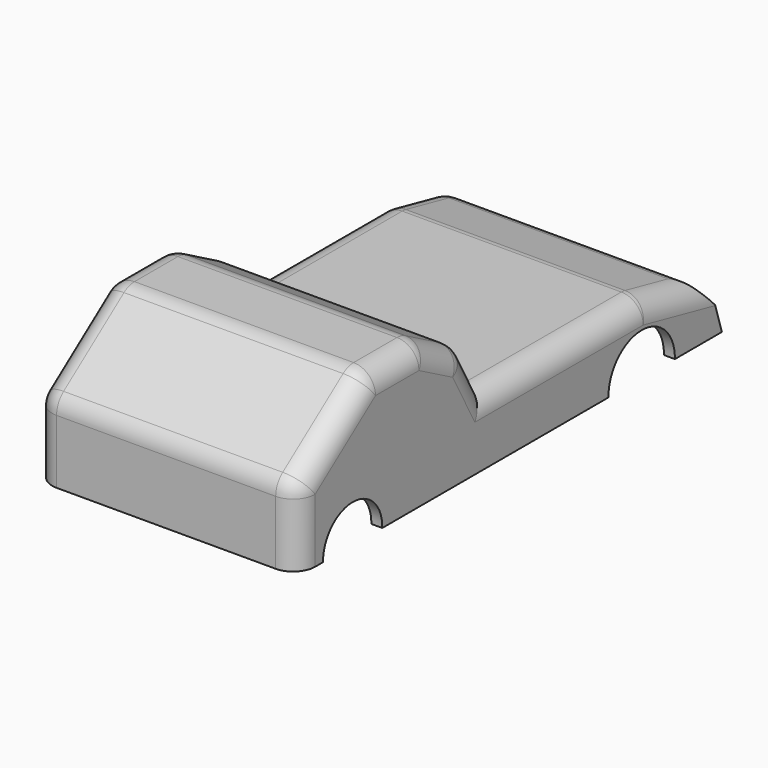
from build123d import *

# Parameters (mm, degrees)
F1_DEPTH      = 60
F2_T          = -2.5
F3_T1_DEPTH   = 31.5029107171
F3_T3_DEPTH   = 19.2704775269
F3_T5_DEPTH   = 59.0151251094
F3_T7_DEPTH   = 50
F3_T9_DEPTH   = 12.544705842
F3_T11_DEPTH  = 26.6507558857
F3_T13_DEPTH  = 10.9735782615
F3_T15_DEPTH  = 12.384029335
F3_T17_DEPTH  = 21.4746284083
F3_T19_DEPTH  = 27.0595039158
F3_T24_DEPTH  = 5
F3_T30_DEPTH  = 5
F3_T36_DEPTH  = 5
F3_T42_DEPTH  = 5
F3_T48_DEPTH  = 5
F3_T54_DEPTH  = 5
F3_T60_DEPTH  = 5
F3_T66_DEPTH  = 5
F3_T72_DEPTH  = 5
F3_T78_DEPTH  = 5
F3_T84_DEPTH  = 5
F3_T90_DEPTH  = 57.5475311177
F3_T95_DEPTH  = 22.7575976563
F3_T100_DEPTH = 57.5475311177
F3_T105_DEPTH = 22.7575976563
F3_T111_DEPTH = 22.7575976563
F3_T115_DEPTH = 57.5475311177
F3_T122_DEPTH = 57.5475311177
F3_T126_DEPTH = 22.7575976563
F4_R          = 8.968677233
F4_R_2        = 8.5168287605
F5_DEPTH      = 60
F6_R          = 9.472590991
F6_R_2        = 8.4503132789
F7_DEPTH      = 65.4


# Not quite as in the source:
# - a fillet or chamfer that OpenCascade refuses, or shapes differently, is made with other operations: its cross-section is extruded or revolved along the edge and cut away or added


with BuildPart() as f1:
    # F0 (on Right) → F1 (new body)
    with BuildSketch(Plane.YZ):
        Polygon((-44.8060370982, 22.3060343415), (-65.3663799167, 6.9827586412), (-65.3663799167, -10.0862076506), (55.6681081653, -10.0862076506), (53.7284500897, -3.8793103304), (48.1034480035, 2.3275862914), (33.7500013411, 5.4310346022), (20.5603465438, 5.4310346022), (4.4612074271, 5.4310346022), (-11.8318963796, 5.4310346022), (-17.4568966031, 15.7112069428), (-29.4827595353, 22.3060343415), align=None)
    extrude(amount=F1_DEPTH)

    # F2
    f2_openings = [f1.faces().sort_by_distance(p)[0] for p in [
        (30, -4.849136, -10.086208),
    ]]
    offset(amount=F2_T, openings=f2_openings, kind=Kind.INTERSECTION)

    # F3: fillet of radius 5 on 22 edges, made by hand

    # F3_s2 → F3_t1 (cut)
    with BuildSketch(Plane(origin=(0, 11.5526545627, -36.9684438457), x_dir=(1, 0, 0), z_dir=(0, -0.2982753662, 0.9544798614))):
        with BuildLine():
            ThreePointArc((5, 50.125620888), (1.4644660941, 48.661154794), (0, 45.125620888))
            Line((0, 45.125620888), (0, 50.125620888))
            Line((0, 50.125620888), (5, 50.125620888))
        make_face()
    extrude(amount=F3_T1_DEPTH, mode=Mode.SUBTRACT)

    # F3_s4 → F3_t3 (cut)
    with BuildSketch(Plane(origin=(0, 34.5525169769, -38.1269015747), x_dir=(1, 0, 0), z_dir=(0, -0.6715195573, 0.7409868313))):
        with BuildLine():
            ThreePointArc((5, 37.2070412259), (1.4644660941, 35.7425751318), (0, 32.2070412259))
            Line((0, 32.2070412259), (0, 37.2070412259))
            Line((0, 37.2070412259), (5, 37.2070412259))
        make_face()
    extrude(amount=F3_T3_DEPTH, mode=Mode.SUBTRACT)

    # F3_s6 → F3_t5 (cut)
    with BuildSketch(Plane.YZ.offset(5)):
        with BuildLine():
            ThreePointArc((46.533671949, 2.6669973721), (47.9776130651, 2.1097041201), (49.1819420179, 1.1375243586))
            Line((49.1819420179, 1.1375243586), (48.1034480035, 2.3275862914))
            Line((48.1034480035, 2.3275862914), (46.533671949, 2.6669973721))
        make_face()
    extrude(amount=F3_T5_DEPTH, mode=Mode.SUBTRACT)

    # F3_s8 → F3_t7 (cut)
    with BuildSketch(Plane.YZ.offset(5)):
        with BuildLine():
            ThreePointArc((33.2156347381, 5.4310346022), (33.7469754945, 5.4027221427), (34.2722988256, 5.3181054024))
            Line((34.2722988256, 5.3181054024), (33.7500013411, 5.4310346022))
            Line((33.7500013411, 5.4310346022), (33.2156347381, 5.4310346022))
        make_face()
        with BuildLine():
            ThreePointArc((-46.1356544501, 21.3150930211), (-44.7217318567, 22.051837403), (-43.147770834, 22.3060343415))
            Line((-43.147770834, 22.3060343415), (-44.8060370982, 22.3060343415))
            Line((-44.8060370982, 22.3060343415), (-46.1356544501, 21.3150930211))
        make_face()
        with BuildLine():
            ThreePointArc((-63.3542635327, 8.4823549449), (-64.8351279561, 6.7161272798), (-65.3663799167, 4.4732962652))
            Line((-65.3663799167, 4.4732962652), (-65.3663799167, 6.9827586412))
            Line((-65.3663799167, 6.9827586412), (-63.3542635327, 8.4823549449))
        make_face()
        with BuildLine():
            ThreePointArc((-28.3595786282, 21.6900964864), (-29.5228367333, 22.1496027948), (-30.763741499, 22.3060343415))
            Line((-30.763741499, 22.3060343415), (-29.4827595353, 22.3060343415))
            Line((-29.4827595353, 22.3060343415), (-28.3595786282, 21.6900964864))
        make_face()
        with BuildLine():
            ThreePointArc((-18.7378088181, 16.4136426032), (-17.604783068, 15.5634588744), (-16.7556605267, 14.4296376218))
            Line((-16.7556605267, 14.4296376218), (-17.4568966031, 15.7112069428))
            Line((-17.4568966031, 15.7112069428), (-18.7378088181, 16.4136426032))
        make_face()
    extrude(amount=F3_T7_DEPTH, mode=Mode.SUBTRACT)

    # F3_s10 → F3_t9 (cut)
    with BuildSketch(Plane(origin=(0, 43.9045114329, -9.492868511), x_dir=(1, 0, 0), z_dir=(0, -0.97741416, 0.2113328175))):
        with BuildLine():
            ThreePointArc((5, 12.4408529979), (1.4644660941, 10.9763869038), (0, 7.4408529979))
            Line((0, 7.4408529979), (0, 12.4408529979))
            Line((0, 12.4408529979), (5, 12.4408529979))
        make_face()
    extrude(amount=F3_T9_DEPTH, mode=Mode.SUBTRACT)

    # F3_s12 → F3_t11 (cut)
    with BuildSketch(Plane(origin=(0, 57.6919644879, -12.4739398105), x_dir=(1, 0, 0), z_dir=(0, -0.97741416, 0.2113328175))):
        with BuildLine():
            ThreePointArc((60, 7.4408529979), (58.5355339059, 10.9763869038), (55, 12.4408529979))
            Line((55, 12.4408529979), (60, 12.4408529979))
            Line((60, 12.4408529979), (60, 7.4408529979))
        make_face()
    extrude(amount=F3_T11_DEPTH, mode=Mode.SUBTRACT)

    # F3_s14 → F3_t13 (cut)
    with BuildSketch(Plane(origin=(0, -21.3256194356, 11.6946933572), x_dir=(1, 0, 0), z_dir=(0, -0.876812429, 0.4808325742))):
        with BuildLine():
            ThreePointArc((5, 5.3819369913), (1.4644660941, 3.9174708973), (0, 0.3819369913))
            Line((0, 0.3819369913), (0, 5.3819369913))
            Line((0, 5.3819369913), (5, 5.3819369913))
        make_face()
        with BuildLine():
            ThreePointArc((60, 0.3819369913), (58.5355339059, 3.9174708973), (55, 5.3819369913))
            Line((55, 5.3819369913), (60, 5.3819369913))
            Line((60, 5.3819369913), (60, 0.3819369913))
        make_face()
    extrude(amount=F3_T13_DEPTH, mode=Mode.SUBTRACT)

    # F3_s16 → F3_t15 (cut)
    with BuildSketch(Plane.XZ.offset(30.763741499)):
        with BuildLine():
            ThreePointArc((0, 17.3060343415), (1.4644660941, 20.8415682474), (5, 22.3060343415))
            Line((5, 22.3060343415), (0, 22.3060343415))
            Line((0, 22.3060343415), (0, 17.3060343415))
        make_face()
        with BuildLine():
            ThreePointArc((60, 17.3060343415), (58.5355339059, 20.8415682474), (55, 22.3060343415))
            Line((55, 22.3060343415), (60, 22.3060343415))
            Line((60, 22.3060343415), (60, 17.3060343415))
        make_face()
    extrude(amount=F3_T15_DEPTH, mode=Mode.SUBTRACT)

    # F3_s18 → F3_t17 (cut)
    with BuildSketch(Plane(origin=(0, -19.4477077147, -14.4940475789), x_dir=(1, 0, 0), z_dir=(0, -0.8018117359, -0.5975767232))):
        with BuildLine():
            ThreePointArc((5, 44.660284946), (1.4644660941, 43.195818852), (0, 39.660284946))
            Line((0, 39.660284946), (0, 44.660284946))
            Line((0, 44.660284946), (5, 44.660284946))
        make_face()
        with BuildLine():
            ThreePointArc((55, 44.660284946), (58.5355339059, 43.195818852), (60, 39.660284946))
            Line((60, 39.660284946), (60, 44.660284946))
            Line((60, 44.660284946), (55, 44.660284946))
        make_face()
    extrude(amount=F3_T17_DEPTH, mode=Mode.SUBTRACT)

    # F3_s20 → F3_t19 (cut)
    with BuildSketch(Plane.XY.offset(-22.5862076506)):
        with BuildLine():
            ThreePointArc((0, -60.3663799167), (1.4644660941, -63.9019138226), (5, -65.3663799167))
            Line((5, -65.3663799167), (0, -65.3663799167))
            Line((0, -65.3663799167), (0, -60.3663799167))
        make_face()
        with BuildLine():
            ThreePointArc((60, -60.3663799167), (58.5355339059, -63.9019138226), (55, -65.3663799167))
            Line((55, -65.3663799167), (60, -65.3663799167))
            Line((60, -65.3663799167), (60, -60.3663799167))
        make_face()
    extrude(amount=F3_T19_DEPTH, mode=Mode.SUBTRACT)


with BuildPart() as f3_tool22:
    # F3_s23 → F3_t24 (new body)
    with BuildSketch(Plane.YZ.offset(5)):
        Polygon((45.4770078615, -2.2200734281), (46.533671949, 2.6669973721), (48.1034480035, 2.3275862914), (49.1819420179, 1.1375243586), align=None)
    extrude(amount=-F3_T24_DEPTH)

    # F3_s25 → F3_t26 (revolve, cut)
    with BuildSketch(Plane(origin=(5, 45.4770078615, -2.2200734281), x_dir=(0, -0.5001210407, -0.8659555096), z_dir=(0, 0.8659555096, -0.5001210407))):
        with BuildLine():
            ThreePointArc((0, -5), (5, 0), (0, 5))
            Line((0, 5), (0, -5))
        make_face()
    revolve(axis=Axis((5, 45.4770078615, -2.2200734281), (-1, 0, 0)), mode=Mode.SUBTRACT)


with BuildPart() as f1_1:
    add(f1.part)

    # F3_t21: cut F3_tool22
    add(f3_tool22.part, mode=Mode.SUBTRACT)


with BuildPart() as f3_tool28:
    # F3_s29 → F3_t30 (new body)
    with BuildSketch(Plane.YZ.offset(5)):
        Polygon((33.2156347381, 0.4310346022), (33.2156347381, 5.4310346022), (33.7500013411, 5.4310346022), (34.2722988256, 5.3181054024), align=None)
    extrude(amount=-F3_T30_DEPTH)

    # F3_s31 → F3_t32 (revolve, cut)
    with BuildSketch(Plane(origin=(5, 33.2156347381, 0.4310346022), x_dir=(0, -0.1062681513, -0.9943375081), z_dir=(0, 0.9943375081, -0.1062681513))):
        with BuildLine():
            ThreePointArc((0, -5), (5, 0), (0, 5))
            Line((0, 5), (0, -5))
        make_face()
    revolve(axis=Axis((5, 33.2156347381, 0.4310346022), (-1, 0, 0)), mode=Mode.SUBTRACT)


with BuildPart() as f1_2:
    add(f1_1.part)

    # F3_t27: cut F3_tool28
    add(f3_tool28.part, mode=Mode.SUBTRACT)


with BuildPart() as f3_tool34:
    # F3_s35 → F3_t36 (new body)
    with BuildSketch(Plane.YZ.offset(55)):
        Polygon((33.2156347381, 0.4310346022), (33.2156347381, 5.4310346022), (33.7500013411, 5.4310346022), (34.2722988256, 5.3181054024), align=None)
    extrude(amount=F3_T36_DEPTH)

    # F3_s37 → F3_t38 (revolve, cut)
    with BuildSketch(Plane(origin=(55, 33.2156347381, 0.4310346022), x_dir=(0, -0.1062681513, -0.9943375081), z_dir=(0, -0.9943375081, 0.1062681513))):
        with BuildLine():
            ThreePointArc((0, -5), (5, 0), (0, 5))
            Line((0, 5), (0, -5))
        make_face()
    revolve(axis=Axis((55, 33.2156347381, 0.4310346022), (1, 0, 0)), mode=Mode.SUBTRACT)


with BuildPart() as f1_3:
    add(f1_2.part)

    # F3_t33: cut F3_tool34
    add(f3_tool34.part, mode=Mode.SUBTRACT)


with BuildPart() as f3_tool40:
    # F3_s41 → F3_t42 (new body)
    with BuildSketch(Plane.YZ.offset(5)):
        Polygon((-21.1419716889, 12.0295804583), (-18.7378088181, 16.4136426032), (-17.4568966031, 15.7112069428), (-16.7556605267, 14.4296376218), align=None)
    extrude(amount=-F3_T42_DEPTH)

    # F3_s43 → F3_t44 (revolve, cut)
    with BuildSketch(Plane(origin=(5, -21.1419716889, 12.0295804583), x_dir=(0, -0.7074377242, -0.7067756832), z_dir=(0, 0.7067756832, -0.7074377242))):
        with BuildLine():
            ThreePointArc((0, -5), (5, 0), (0, 5))
            Line((0, 5), (0, -5))
        make_face()
    revolve(axis=Axis((5, -21.1419716889, 12.0295804583), (-1, 0, 0)), mode=Mode.SUBTRACT)


with BuildPart() as f1_4:
    add(f1_3.part)

    # F3_t39: cut F3_tool40
    add(f3_tool40.part, mode=Mode.SUBTRACT)


with BuildPart() as f3_tool46:
    # F3_s47 → F3_t48 (new body)
    with BuildSketch(Plane.YZ.offset(5)):
        Polygon((-30.763741499, 17.3060343415), (-28.3595786282, 21.6900964864), (-29.4827595353, 22.3060343415), (-30.763741499, 22.3060343415), align=None)
    extrude(amount=-F3_T48_DEPTH)

    # F3_s49 → F3_t50 (revolve, cut)
    with BuildSketch(Plane(origin=(5, -30.763741499, 17.3060343415), x_dir=(0, -0.2481809531, -0.9687136907), z_dir=(0, 0.9687136907, -0.2481809531))):
        with BuildLine():
            ThreePointArc((0, -5), (5, 0), (0, 5))
            Line((0, 5), (0, -5))
        make_face()
    revolve(axis=Axis((5, -30.763741499, 17.3060343415), (-1, 0, 0)), mode=Mode.SUBTRACT)


with BuildPart() as f1_5:
    add(f1_4.part)

    # F3_t45: cut F3_tool46
    add(f3_tool46.part, mode=Mode.SUBTRACT)


with BuildPart() as f3_tool52:
    # F3_s53 → F3_t54 (new body)
    with BuildSketch(Plane.YZ.offset(5)):
        Polygon((-43.147770834, 17.3060343415), (-46.1356544501, 21.3150930211), (-44.8060370982, 22.3060343415), (-43.147770834, 22.3060343415), align=None)
    extrude(amount=-F3_T54_DEPTH)

    # F3_s55 → F3_t56 (revolve, cut)
    with BuildSketch(Plane(origin=(5, -43.147770834, 17.3060343415), x_dir=(0, 0.3147922045, -0.9491606123), z_dir=(0, 0.9491606123, 0.3147922045))):
        with BuildLine():
            ThreePointArc((0, -5), (5, 0), (0, 5))
            Line((0, 5), (0, -5))
        make_face()
    revolve(axis=Axis((5, -43.147770834, 17.3060343415), (-1, 0, 0)), mode=Mode.SUBTRACT)


with BuildPart() as f1_6:
    add(f1_5.part)

    # F3_t51: cut F3_tool52
    add(f3_tool52.part, mode=Mode.SUBTRACT)


with BuildPart() as f3_tool58:
    # F3_s59 → F3_t60 (new body)
    with BuildSketch(Plane.YZ.offset(5)):
        Polygon((-60.3663799167, 4.4732962652), (-65.3663799167, 4.4732962652), (-65.3663799167, 6.9827586412), (-63.3542635327, 8.4823549449), align=None)
    extrude(amount=-F3_T60_DEPTH)

    # F3_s61 → F3_t62 (revolve, cut)
    with BuildSketch(Plane(origin=(5, -60.3663799167, 4.4732962652), x_dir=(0, 0.8937496079, -0.4485662029), z_dir=(0, 0.4485662029, 0.8937496079))):
        with BuildLine():
            ThreePointArc((0, -5), (5, 0), (0, 5))
            Line((0, 5), (0, -5))
        make_face()
    revolve(axis=Axis((5, -60.3663799167, 4.4732962652), (-1, 0, 0)), mode=Mode.SUBTRACT)


with BuildPart() as f1_7:
    add(f1_6.part)

    # F3_t57: cut F3_tool58
    add(f3_tool58.part, mode=Mode.SUBTRACT)


with BuildPart() as f3_tool64:
    # F3_s65 → F3_t66 (new body)
    with BuildSketch(Plane.YZ.offset(55)):
        Polygon((-21.1419716889, 12.0295804583), (-18.7378088181, 16.4136426032), (-17.4568966031, 15.7112069428), (-16.7556605267, 14.4296376218), align=None)
    extrude(amount=F3_T66_DEPTH)

    # F3_s67 → F3_t68 (revolve, cut)
    with BuildSketch(Plane(origin=(55, -21.1419716889, 12.0295804583), x_dir=(0, -0.7074377242, -0.7067756832), z_dir=(0, -0.7067756832, 0.7074377242))):
        with BuildLine():
            ThreePointArc((0, -5), (5, 0), (0, 5))
            Line((0, 5), (0, -5))
        make_face()
    revolve(axis=Axis((55, -21.1419716889, 12.0295804583), (1, 0, 0)), mode=Mode.SUBTRACT)


with BuildPart() as f1_8:
    add(f1_7.part)

    # F3_t63: cut F3_tool64
    add(f3_tool64.part, mode=Mode.SUBTRACT)


with BuildPart() as f3_tool70:
    # F3_s71 → F3_t72 (new body)
    with BuildSketch(Plane.YZ.offset(55)):
        Polygon((-30.763741499, 17.3060343415), (-28.3595786282, 21.6900964864), (-29.4827595353, 22.3060343415), (-30.763741499, 22.3060343415), align=None)
    extrude(amount=F3_T72_DEPTH)

    # F3_s73 → F3_t74 (revolve, cut)
    with BuildSketch(Plane(origin=(55, -30.763741499, 17.3060343415), x_dir=(0, -0.2481809531, -0.9687136907), z_dir=(0, -0.9687136907, 0.2481809531))):
        with BuildLine():
            ThreePointArc((0, -5), (5, 0), (0, 5))
            Line((0, 5), (0, -5))
        make_face()
    revolve(axis=Axis((55, -30.763741499, 17.3060343415), (1, 0, 0)), mode=Mode.SUBTRACT)


with BuildPart() as f1_9:
    add(f1_8.part)

    # F3_t69: cut F3_tool70
    add(f3_tool70.part, mode=Mode.SUBTRACT)


with BuildPart() as f3_tool76:
    # F3_s77 → F3_t78 (new body)
    with BuildSketch(Plane.YZ.offset(55)):
        Polygon((-43.147770834, 17.3060343415), (-43.147770834, 22.3060343415), (-44.8060370982, 22.3060343415), (-46.1356544501, 21.3150930211), align=None)
    extrude(amount=F3_T78_DEPTH)

    # F3_s79 → F3_t80 (revolve, cut)
    with BuildSketch(Plane(origin=(55, -43.147770834, 17.3060343415), x_dir=(0, 0.3147922045, -0.9491606123), z_dir=(0, -0.9491606123, -0.3147922045))):
        with BuildLine():
            ThreePointArc((0, -5), (5, 0), (0, 5))
            Line((0, 5), (0, -5))
        make_face()
    revolve(axis=Axis((55, -43.147770834, 17.3060343415), (1, 0, 0)), mode=Mode.SUBTRACT)


with BuildPart() as f1_10:
    add(f1_9.part)

    # F3_t75: cut F3_tool76
    add(f3_tool76.part, mode=Mode.SUBTRACT)


with BuildPart() as f3_tool82:
    # F3_s83 → F3_t84 (new body)
    with BuildSketch(Plane.YZ.offset(55)):
        Polygon((-60.3663799167, 4.4732962652), (-65.3663799167, 4.4732962652), (-65.3663799167, 6.9827586412), (-63.3542635327, 8.4823549449), align=None)
    extrude(amount=F3_T84_DEPTH)

    # F3_s85 → F3_t86 (revolve, cut)
    with BuildSketch(Plane(origin=(55, -60.3663799167, 4.4732962652), x_dir=(0, 0.8937496079, -0.4485662029), z_dir=(0, -0.4485662029, -0.8937496079))):
        with BuildLine():
            ThreePointArc((0, -5), (5, 0), (0, 5))
            Line((0, 5), (0, -5))
        make_face()
    revolve(axis=Axis((55, -60.3663799167, 4.4732962652), (1, 0, 0)), mode=Mode.SUBTRACT)


with BuildPart() as f1_11:
    add(f1_10.part)

    # F3_t81: cut F3_tool82
    add(f3_tool82.part, mode=Mode.SUBTRACT)


with BuildPart() as f3_tool88:
    # F3_s89 → F3_t90 (new body)
    with BuildSketch(Plane.XZ.offset(-33.2156347381)):
        with BuildLine():
            ThreePointArc((5, 5.4310346022), (1.4644660941, 3.9665685082), (0, 0.4310346022))
            Line((0, 0.4310346022), (0, 5.4310346022))
            Line((0, 5.4310346022), (5, 5.4310346022))
        make_face()
    extrude(amount=F3_T90_DEPTH)

    split(bisect_by=Plane(origin=(0, -6.818711183, -3.7309930863), x_dir=(1, 0, 0), z_dir=(0, 0.8772622324, 0.4800114327)), keep=Keep.TOP)


with BuildPart() as f1_12:
    add(f1_11.part)

    # F3_t87: cut F3_tool88
    add(f3_tool88.part, mode=Mode.SUBTRACT)


with BuildPart() as f3_tool93:
    # F3_s94 → F3_t95 (new body)
    with BuildSketch(Plane(origin=(0, 0.9869577122, -1.8037502171), x_dir=(1, 0, 0), z_dir=(0, -0.4800114327, 0.8772622324))):
        with BuildLine():
            ThreePointArc((5, -7.7727171316), (1.4644660941, -9.2371832257), (0, -12.7727171316))
            Line((0, -12.7727171316), (0, -7.7727171316))
            Line((0, -7.7727171316), (5, -7.7727171316))
        make_face()
    extrude(amount=F3_T95_DEPTH)

    split(bisect_by=Plane.XY.offset(5.4310346022), keep=Keep.TOP)


with BuildPart() as f1_13:
    add(f1_12.part)

    # F3_t92: cut F3_tool93
    add(f3_tool93.part, mode=Mode.SUBTRACT)


with BuildPart() as f3_tool98:
    # F3_s99 → F3_t100 (new body)
    with BuildSketch(Plane.XZ.offset(24.3318963796)):
        with BuildLine():
            ThreePointArc((60, 0.4310346022), (58.5355339059, 3.9665685082), (55, 5.4310346022))
            Line((55, 5.4310346022), (60, 5.4310346022))
            Line((60, 5.4310346022), (60, 0.4310346022))
        make_face()
    extrude(amount=-F3_T100_DEPTH)

    split(bisect_by=Plane(origin=(0, -6.818711183, -3.7309930863), x_dir=(1, 0, 0), z_dir=(0, 0.8772622324, 0.4800114327)), keep=Keep.TOP)


with BuildPart() as f1_14:
    add(f1_13.part)

    # F3_t97: cut F3_tool98
    add(f3_tool98.part, mode=Mode.SUBTRACT)


with BuildPart() as f3_tool103:
    # F3_s104 → F3_t105 (new body)
    with BuildSketch(Plane(origin=(0, 0.9869577122, -1.8037502171), x_dir=(1, 0, 0), z_dir=(0, -0.4800114327, 0.8772622324))):
        with BuildLine():
            ThreePointArc((60, -12.7727171316), (58.5355339059, -9.2371832257), (55, -7.7727171316))
            Line((55, -7.7727171316), (60, -7.7727171316))
            Line((60, -7.7727171316), (60, -12.7727171316))
        make_face()
    extrude(amount=F3_T105_DEPTH)

    split(bisect_by=Plane.XY.offset(5.4310346022), keep=Keep.TOP)


with BuildPart() as f1_15:
    add(f1_14.part)

    # F3_t102: cut F3_tool103
    add(f3_tool103.part, mode=Mode.SUBTRACT)


with BuildPart() as f3_tool109:
    # F3_s110 → F3_t111 (new body)
    with BuildSketch(Plane(origin=(0, 0.9869577122, -1.8037502171), x_dir=(1, 0, 0), z_dir=(0, -0.4800114327, 0.8772622324))):
        with BuildLine():
            ThreePointArc((5, -7.7727171316), (1.4644660941, -9.2371832257), (0, -12.7727171316))
            Line((0, -12.7727171316), (0, -7.7727171316))
            Line((0, -7.7727171316), (5, -7.7727171316))
        make_face()
    extrude(amount=F3_T111_DEPTH)

    split(bisect_by=Plane.XY.offset(5.4310346022), keep=Keep.BOTTOM)


with BuildPart() as f3_tool113:
    # F3_s114 → F3_t115 (new body)
    with BuildSketch(Plane.XZ.offset(-33.2156347381)):
        with BuildLine():
            ThreePointArc((5, 5.4310346022), (1.4644660941, 3.9665685082), (0, 0.4310346022))
            Line((0, 0.4310346022), (0, 5.4310346022))
            Line((0, 5.4310346022), (5, 5.4310346022))
        make_face()
    extrude(amount=F3_T115_DEPTH)

    split(bisect_by=Plane(origin=(0, -6.818711183, -3.7309930863), x_dir=(1, 0, 0), z_dir=(0, -0.8772622324, -0.4800114327)), keep=Keep.TOP)


with BuildPart() as f3_tool109_1:
    add(f3_tool109.part)

    # F3_t117: intersect F3_tool113
    add(f3_tool113.part, mode=Mode.INTERSECT)


with BuildPart() as f1_16:
    add(f1_15.part)

    # F3_t107: cut F3_tool109
    add(f3_tool109_1.part, mode=Mode.SUBTRACT)


with BuildPart() as f3_tool120:
    # F3_s121 → F3_t122 (new body)
    with BuildSketch(Plane.XZ.offset(24.3318963796)):
        with BuildLine():
            ThreePointArc((60, 0.4310346022), (58.5355339059, 3.9665685082), (55, 5.4310346022))
            Line((55, 5.4310346022), (60, 5.4310346022))
            Line((60, 5.4310346022), (60, 0.4310346022))
        make_face()
    extrude(amount=-F3_T122_DEPTH)

    split(bisect_by=Plane(origin=(0, -6.818711183, -3.7309930863), x_dir=(1, 0, 0), z_dir=(0, -0.8772622324, -0.4800114327)), keep=Keep.TOP)


with BuildPart() as f3_tool124:
    # F3_s125 → F3_t126 (new body)
    with BuildSketch(Plane(origin=(0, 0.9869577122, -1.8037502171), x_dir=(1, 0, 0), z_dir=(0, -0.4800114327, 0.8772622324))):
        with BuildLine():
            ThreePointArc((60, -12.7727171316), (58.5355339059, -9.2371832257), (55, -7.7727171316))
            Line((55, -7.7727171316), (60, -7.7727171316))
            Line((60, -7.7727171316), (60, -12.7727171316))
        make_face()
    extrude(amount=F3_T126_DEPTH)

    split(bisect_by=Plane.XY.offset(5.4310346022), keep=Keep.BOTTOM)


with BuildPart() as f3_tool120_1:
    add(f3_tool120.part)

    # F3_t128: intersect F3_tool124
    add(f3_tool124.part, mode=Mode.INTERSECT)


with BuildPart() as f1_17:
    add(f1_16.part)

    # F3_t118: cut F3_tool120
    add(f3_tool120_1.part, mode=Mode.SUBTRACT)

    # F4 (on Right) → F5 (cut)
    with BuildSketch(Plane.YZ):
        with Locations((33.9439660311, -9.892241098)):
            Circle(F4_R)
        with Locations((-48.2974201441, -9.698276408)):
            Circle(F4_R_2)
    extrude(amount=-F5_DEPTH, mode=Mode.SUBTRACT)

    # F6 (on Right) → F7 (cut)
    with BuildSketch(Plane.YZ):
        with Locations((32.780174166, -9.892241098)):
            Circle(F6_R)
        with Locations((-49.6551729739, -9.892241098)):
            Circle(F6_R_2)
    extrude(amount=F7_DEPTH, mode=Mode.SUBTRACT)


solid = f1_17.part
